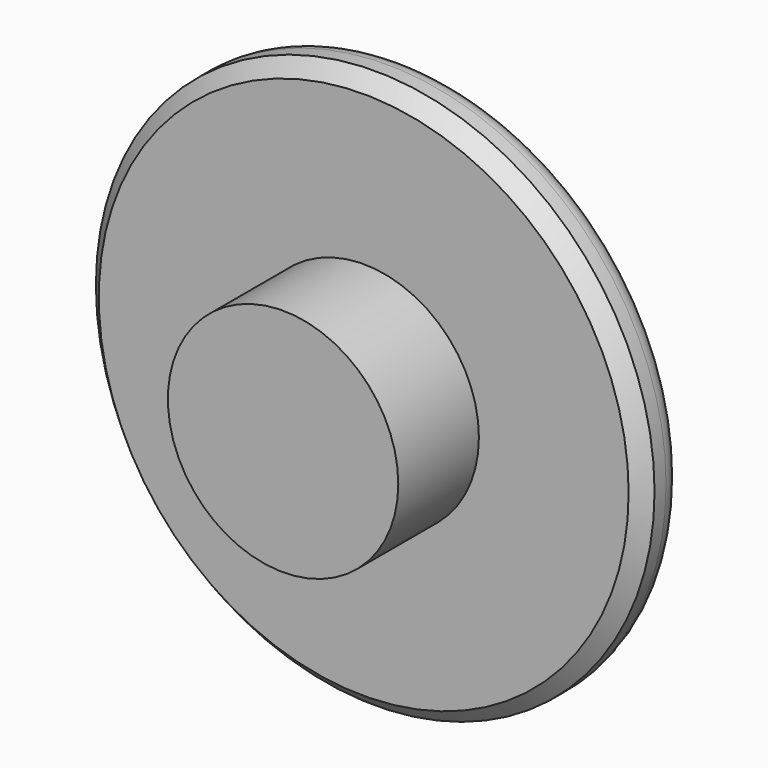
from build123d import *

# Parameters (mm, degrees)
F0_R     = 4
F1_DEPTH = 5.25
F0_R_2   = 9.7
F2_DEPTH = 1.75
F3_SIZE  = 0.5
F4_R     = 0.75


# Not quite as in the source:
# - a feature names something its author has since deleted; it is built from what else it names


with BuildPart() as f1:
    # F0 (on Front) → F1 (new body)
    with BuildSketch(Plane.XZ):
        Circle(F0_R)
    extrude(amount=F1_DEPTH)

    # F0 (on Front) → F2 (join)
    with BuildSketch(Plane.XZ):
        Circle(F0_R_2)
        Circle(F0_R, mode=Mode.SUBTRACT)
    extrude(amount=F2_DEPTH)

    # F3
    f3_edges = [f1.edges().sort_by_distance(p)[0] for p in [
        (-9.7, -1.75, 0),
    ]]
    chamfer(f3_edges, length=F3_SIZE)

    # F4
    f4_edges = [f1.edges().sort_by_distance(p)[0] for p in [
        (-9.7, 0, 0),
    ]]
    fillet(f4_edges, radius=F4_R)


solid = f1.part
